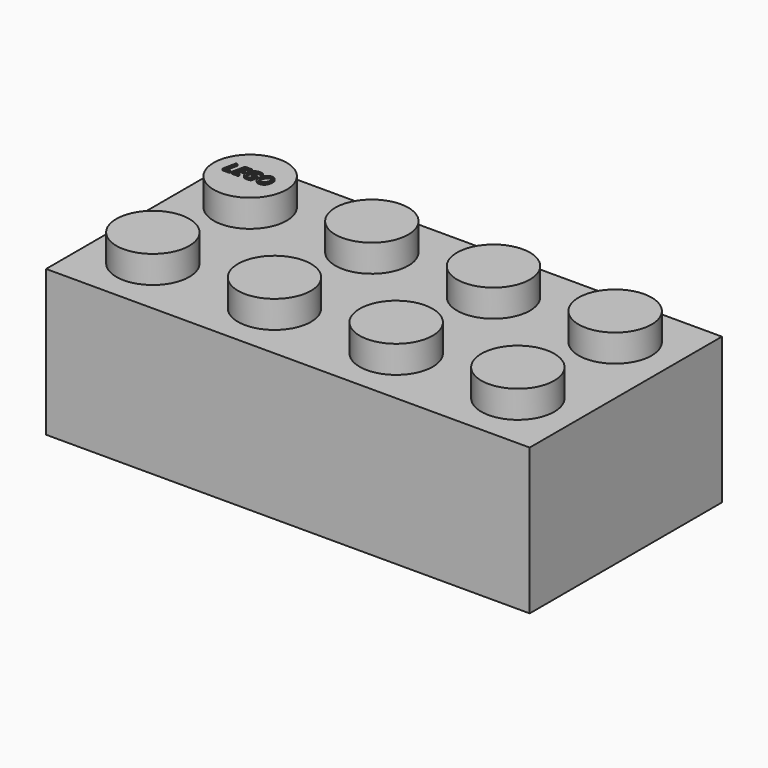
from build123d import *

# Parameters (mm, degrees)
F4_W          = 31.8
F4_H          = 15.8
F4_R          = 2.4
F5_DEPTH      = 9.6
F6_T          = -1.5
F7_DEPTH      = 1.8
F8_R          = 3.255
F8_R_2        = 2.4
F9_DEPTH      = 8.1
F10_TEXT_SIZE = 1.2418342927
F11_DEPTH     = 0.1


# Not quite as in the source:
# - Text() gives the source's letters only with a copy of the font that has no kerning and outlines rounded to 1/6400 em; it was checked with that copy


with BuildPart() as f5:
    # F4 (on Top) → F5 (new body)
    with BuildSketch(Plane.XY):
        Rectangle(F4_W, F4_H)
        with Locations((-12, -4)):
            Circle(F4_R, mode=Mode.SUBTRACT)
        with Locations((-4, -4)):
            Circle(F4_R, mode=Mode.SUBTRACT)
        with Locations((4, -4)):
            Circle(F4_R, mode=Mode.SUBTRACT)
        with Locations((12, -4)):
            Circle(F4_R, mode=Mode.SUBTRACT)
        with Locations((-12, 4)):
            Circle(F4_R, mode=Mode.SUBTRACT)
        with Locations((-4, 4)):
            Circle(F4_R, mode=Mode.SUBTRACT)
        with Locations((4, 4)):
            Circle(F4_R, mode=Mode.SUBTRACT)
        with Locations((12, 4)):
            Circle(F4_R, mode=Mode.SUBTRACT)
        with Locations((-12, 4)):
            Circle(F4_R)
        with Locations((-4, 4)):
            Circle(F4_R)
        with Locations((4, 4)):
            Circle(F4_R)
        with Locations((12, 4)):
            Circle(F4_R)
        with Locations((12, -4)):
            Circle(F4_R)
        with Locations((4, -4)):
            Circle(F4_R)
        with Locations((-4, -4)):
            Circle(F4_R)
        with Locations((-12, -4)):
            Circle(F4_R)
    extrude(amount=-F5_DEPTH)

    # F6
    f6_openings = [f5.faces().sort_by_distance(p)[0] for p in [
        (0, 0, -9.6),
    ]]
    offset(amount=F6_T, openings=f6_openings)

    # F4 (on Top) → F7 (join)
    with BuildSketch(Plane.XY):
        with Locations((-12, -4)):
            Circle(F4_R)
        with Locations((-12, 4)):
            Circle(F4_R)
        with Locations((-4, 4)):
            Circle(F4_R)
        with Locations((4, 4)):
            Circle(F4_R)
        with Locations((12, 4)):
            Circle(F4_R)
        with Locations((12, -4)):
            Circle(F4_R)
        with Locations((4, -4)):
            Circle(F4_R)
        with Locations((-4, -4)):
            Circle(F4_R)
    extrude(amount=F7_DEPTH)

    # F8 (on face) → F9 (join)
    with BuildSketch(Plane(origin=(0, 0, -1.5), x_dir=(1, 0, 0), z_dir=(0, 0, -1))):
        with Locations((-8, 0)):
            Circle(F8_R)
        with Locations((-8, 0)):
            Circle(F8_R_2, mode=Mode.SUBTRACT)
        Circle(F8_R)
        Circle(F8_R_2, mode=Mode.SUBTRACT)
        with Locations((8, 0)):
            Circle(F8_R)
        with Locations((8, 0)):
            Circle(F8_R_2, mode=Mode.SUBTRACT)
    extrude(amount=F9_DEPTH)

    # F10 (on face) → F11 (join)
    with BuildSketch(Plane.XY.offset(1.8)):
        with Locations((-13.5700851842, 3.6202500544)):
            Text('LEGO', F10_TEXT_SIZE, font='Open Sans', font_style=FontStyle.ITALIC, text_align=(TextAlign.LEFT, TextAlign.BOTTOM))
    extrude(amount=F11_DEPTH)


solid = f5.part
